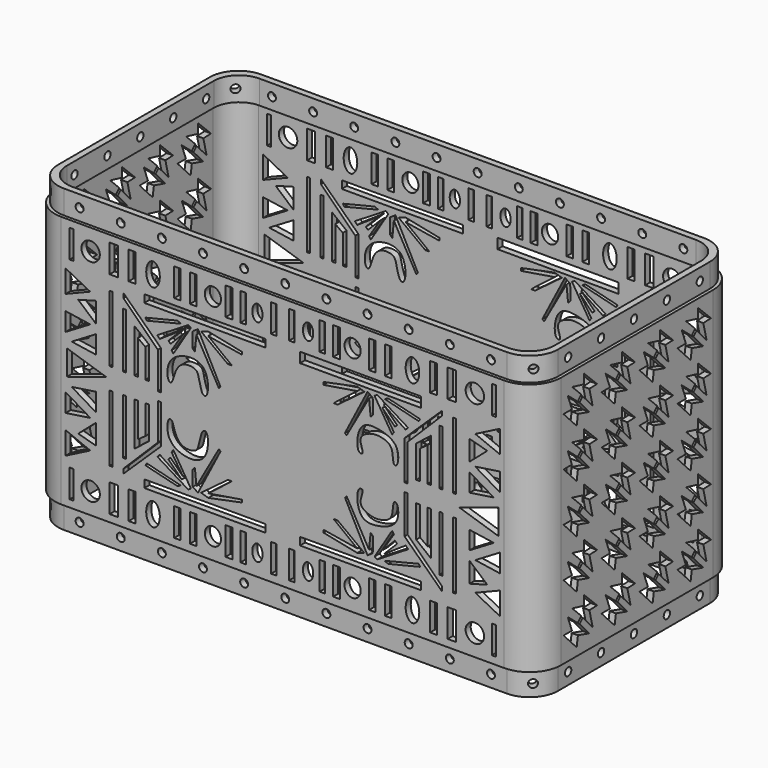
from build123d import *

# Parameters (mm, degrees)
F1_DEPTH  = 101.6
F2_T      = -2.54
F4_DEPTH  = 9.525
F6_DEPTH  = 9.525
F8_W      = 1.27
F8_H      = 26.6622491181
F8_H_2    = 22.2469121218
F8_W_2    = 48.6389496364
F8_H_3    = 3.0932202935
F8_H_4    = 4.0642395616
F8_H_5    = 0.0183284283
F8_H_6    = 3.0748918653
F8_W_3    = 1.6330480576
F8_H_7    = 11.2412478775
F8_R      = 3.7023981113
F8_W_4    = 3.2661110163
F8_W_5    = 2.7217492461
F8_W_6    = 2.6040747762
F8_W_7    = 2.5893896818
F8_W_8    = 2.1774070337
F8_W_9    = 2.7217566967
F8_W_10   = 2.1774061024
F9_DEPTH  = 127
F10_R     = 1.5875
F11_DEPTH = 127
F13_DEPTH = 228.6
F14_R     = 1.5875
F15_DEPTH = 228.6
F17_R     = 1.5875
F18_DEPTH = 50.8
F21_R     = 1.5875
F22_DEPTH = 50.8
F24_R     = 1.5875
F25_DEPTH = 76.2
F27_R     = 1.5875
F28_DEPTH = 76.2


with BuildPart() as f1:
    # F0 (on Top) → F1 (new body)
    with BuildSketch(Plane.XY):
        with BuildLine():
            Line((88.9, 50.8), (-88.9, 50.8))
            ThreePointArc((-88.9, 50.8), (-97.8802561211, 47.0802561211), (-101.6, 38.1))
            Line((-101.6, 38.1), (-101.6, -38.1))
            ThreePointArc((-101.6, -38.1), (-97.8802561211, -47.0802561211), (-88.9, -50.8))
            Line((-88.9, -50.8), (88.9, -50.8))
            ThreePointArc((88.9, -50.8), (97.8802561211, -47.0802561211), (101.6, -38.1))
            Line((101.6, -38.1), (101.6, 38.1))
            ThreePointArc((101.6, 38.1), (97.8802561211, 47.0802561211), (88.9, 50.8))
        make_face()
    extrude(amount=F1_DEPTH)

    # F2
    f2_openings = [f1.faces().sort_by_distance(p)[0] for p in [
        (0, 0, 101.6),
        (0, 0, 0),
    ]]
    offset(amount=F2_T, openings=f2_openings)

    # F3 (on face) → F4 (join)
    with BuildSketch(Plane.XY.offset(101.6)):
        with BuildLine():
            Line((-88.9, -49.53), (88.9, -49.53))
            ThreePointArc((88.9, -49.53), (96.982230509, -46.182230509), (100.33, -38.1))
            Line((100.33, -38.1), (100.33, 38.1))
            ThreePointArc((100.33, 38.1), (96.982230509, 46.182230509), (88.9, 49.53))
            Line((88.9, 49.53), (-88.9, 49.53))
            ThreePointArc((-88.9, 49.53), (-96.982230509, 46.182230509), (-100.33, 38.1))
            Line((-100.33, 38.1), (-100.33, -38.1))
            ThreePointArc((-100.33, -38.1), (-96.982230509, -46.182230509), (-88.9, -49.53))
        make_face()
        with BuildLine():
            ThreePointArc((-99.06, 38.1), (-96.0842048969, 45.2842048969), (-88.9, 48.26))
            Line((-88.9, 48.26), (88.9, 48.26))
            ThreePointArc((88.9, 48.26), (96.0842048969, 45.2842048969), (99.06, 38.1))
            Line((99.06, 38.1), (99.06, -38.1))
            ThreePointArc((99.06, -38.1), (96.0842048969, -45.2842048969), (88.9, -48.26))
            Line((88.9, -48.26), (-88.9, -48.26))
            ThreePointArc((-88.9, -48.26), (-96.0842048969, -45.2842048969), (-99.06, -38.1))
            Line((-99.06, -38.1), (-99.06, 38.1))
        make_face(mode=Mode.SUBTRACT)
        with BuildLine():
            Line((88.9, 48.26), (-88.9, 48.26))
            ThreePointArc((-88.9, 48.26), (-96.0842048969, 45.2842048969), (-99.06, 38.1))
            Line((-99.06, 38.1), (-99.06, -38.1))
            ThreePointArc((-99.06, -38.1), (-96.0842048969, -45.2842048969), (-88.9, -48.26))
            Line((-88.9, -48.26), (88.9, -48.26))
            ThreePointArc((88.9, -48.26), (96.0842048969, -45.2842048969), (99.06, -38.1))
            Line((99.06, -38.1), (99.06, 38.1))
            ThreePointArc((99.06, 38.1), (96.0842048969, 45.2842048969), (88.9, 48.26))
        make_face()
        with BuildLine():
            ThreePointArc((-97.79, 36.83), (-94.8142048969, 44.0142048969), (-87.63, 46.99))
            Line((-87.63, 46.99), (87.63, 46.99))
            ThreePointArc((87.63, 46.99), (94.8142048969, 44.0142048969), (97.79, 36.83))
            Line((97.79, 36.83), (97.79, -36.83))
            ThreePointArc((97.79, -36.83), (94.8142048969, -44.0142048969), (87.63, -46.99))
            Line((87.63, -46.99), (-87.63, -46.99))
            ThreePointArc((-87.63, -46.99), (-94.8142048969, -44.0142048969), (-97.79, -36.83))
            Line((-97.79, -36.83), (-97.79, 36.83))
        make_face(mode=Mode.SUBTRACT)
    extrude(amount=F4_DEPTH)

    # F5 (on Top) → F6 (join)
    with BuildSketch(Plane.XY):
        with BuildLine():
            Line((88.9, 49.53), (-88.9, 49.53))
            ThreePointArc((-88.9, 49.53), (-96.982230509, 46.182230509), (-100.33, 38.1))
            Line((-100.33, 38.1), (-100.33, -38.1))
            ThreePointArc((-100.33, -38.1), (-96.982230509, -46.182230509), (-88.9, -49.53))
            Line((-88.9, -49.53), (88.9, -49.53))
            ThreePointArc((88.9, -49.53), (96.982230509, -46.182230509), (100.33, -38.1))
            Line((100.33, -38.1), (100.33, 38.1))
            ThreePointArc((100.33, 38.1), (96.982230509, 46.182230509), (88.9, 49.53))
        make_face()
        with BuildLine():
            Line((87.63, -46.99), (-87.63, -46.99))
            ThreePointArc((-87.63, -46.99), (-94.8142048969, -44.0142048969), (-97.79, -36.83))
            Line((-97.79, -36.83), (-97.79, 36.83))
            ThreePointArc((-97.79, 36.83), (-94.8142048969, 44.0142048969), (-87.63, 46.99))
            Line((-87.63, 46.99), (87.63, 46.99))
            ThreePointArc((87.63, 46.99), (94.8142048969, 44.0142048969), (97.79, 36.83))
            Line((97.79, 36.83), (97.79, -36.83))
            ThreePointArc((97.79, -36.83), (94.8142048969, -44.0142048969), (87.63, -46.99))
        make_face(mode=Mode.SUBTRACT)
    extrude(amount=-F6_DEPTH)

    # F8 (on face) → F9 (cut)
    with BuildSketch(Plane.XZ.offset(50.8)):
        with Locations((-68.9020286703, 68.476928398)):
            Rectangle(F8_W, F8_H)
        with Locations((-63.4877477384, 66.1137998104)):
            Rectangle(F8_W, F8_H_2)
        Polygon((-59.5282502472, 72.5896432996), (-59.5282502472, 55.0722591579), (-58.1557303667, 55.0722591579), (-58.1557303667, 68.7985643744), (-55.1492646337, 66.6415765882), (-55.1492646337, 55.0068952143), (-53.5806752741, 55.0068952143), (-53.5806752741, 67.883476615), align=None)
        Polygon((-50.1429028809, 67.2847032547), (-50.1429028809, 52.5627210736), (-48.8572530448, 52.5627210736), (-48.8572530448, 68.2254508138), (-63.9233589172, 82.7843993902), (-63.9233589172, 80.9818580747), align=None)
        with Locations((-31.2301132362, 83.5803337395)):
            Rectangle(F8_W_2, F8_H_3)
        Polygon((-42.2406457365, 80.1282450557), (-55.1029518247, 76.9830867648), (-54.5800887048, 76.0679990053), (-40.8993884921, 79.4538781047), align=None)
        Polygon((-37.9368662834, 79.9399539828), (-50.3318198025, 72.3422840238), (-49.3153783607, 71.3319868494), (-40.5374765396, 77.2372558713), (-45.9055488806, 71.8365368266), (-45.039238331, 70.9754630211), (-40.0128401816, 76.0324299335), (-44.6069753195, 68.9266495444), (-43.8944920897, 67.867577076), (-36.8599989183, 79.27594897), align=None)
        Polygon((-36.1134645205, 78.3830672404), (-36.279860884, 72.3422840238), (-35.2634194421, 71.3319868494), (-34.6407592297, 77.6337906718), (-25.6241530731, 61.6211524411), (-24.9729361385, 62.2763298452), (-34.0206585824, 79.7909870744), align=None)
        Polygon((-32.7727422118, 79.3707743287), (-22.0318287611, 71.3319868494), (-20.3978791833, 71.3319868494), (-29.9133080989, 78.6741450429), (-16.3456853479, 76.4601826668), (-16.3456853479, 77.5059908628), (-29.8969931901, 80.269522965), align=None)
        with BuildLine():
            add(Edge.make_bspline(
                [(-45.6465967, 57.64246732), (-46.3949852869, 58.5152129663), (-46.8754204882, 65.0704943716), (-39.4761129722, 69.4554491147), (-29.7425350447, 68.3388211569), (-29.6427188035, 56.9346913808), (-32.7583018207, 56.9375001196), (-33.6608195324, 63.7843708703), (-35.1035222126, 65.6981368237), (-40.3177607972, 66.1274931074), (-43.3679070085, 62.1610139174), (-44.150056881, 57.2996314955), (-45.3474051799, 57.2935602133), (-45.6465967, 57.64246732)],
                knots=[0, 0, 0, 0, 0.1046718898, 0.2236520347, 0.3429708219, 0.4678825728, 0.5171800771, 0.6233463725, 0.6881859742, 0.7762207213, 0.869134302, 0.9581541697, 1, 1, 1, 1], degree=3))
        make_face()
        Polygon((49.3153783607, 71.3319868494), (50.3318198025, 72.3422840238), (37.9368662834, 79.9399539828), (36.8599989183, 79.27594897), (43.8944920897, 67.867577076), (44.6069753195, 68.9266495444), (40.0128401816, 76.0324299335), (45.039238331, 70.9754630211), (45.9055488806, 71.8365368266), (40.5374765396, 77.2372558713), align=None)
        Polygon((50.1429028809, 67.2847032547), (63.9233589172, 80.9818580747), (63.9233589172, 82.7843993902), (48.8572530448, 68.2254508138), (48.8572530448, 52.5627210736), (50.1429028809, 52.5627210736), align=None)
        Polygon((58.1557303667, 55.0722591579), (59.5282502472, 55.0722591579), (59.5282502472, 72.5896432996), (53.5806752741, 67.883476615), (53.5806752741, 55.0068952143), (55.1492646337, 55.0068952143), (55.1492646337, 66.6415765882), (58.1557303667, 68.7985643744), align=None)
        with Locations((31.2301132362, 83.0948241055)):
            Rectangle(F8_W_2, F8_H_4)
        Polygon((35.2634194421, 71.3319868494), (36.279860884, 72.3422840238), (36.1134645205, 78.3830672404), (34.0206585824, 79.7909870744), (24.9729361385, 62.2763298452), (25.6241530731, 61.6211524411), (34.6407592297, 77.6337906718), align=None)
        Polygon((32.7727422118, 79.3707743287), (29.8969931901, 80.269522965), (16.3456853479, 77.5059908628), (16.3456853479, 76.4601826668), (29.9133080989, 78.6741450429), (20.3978791833, 71.3319868494), (22.0318287611, 71.3319868494), align=None)
        with Locations((63.4877477384, 66.1137998104)):
            Rectangle(F8_W, F8_H_2)
        with Locations((68.9020286703, 68.476928398)):
            Rectangle(F8_W, F8_H)
        Polygon((40.8993884921, 79.4538781047), (54.5800887048, 76.0679990053), (55.1029518247, 76.9830867648), (42.2406457365, 80.1282450557), align=None)
        with BuildLine():
            add(Edge.make_bspline(
                [(45.6465967, 57.64246732), (46.4635562257, 58.5803284783), (47.0830188738, 65.3489604803), (38.5305633944, 68.4932132602), (29.9974402873, 68.4019397724), (29.3300401803, 56.8501614014), (33.1351567804, 57.0444987502), (29.5108019941, 62.8747584858), (35.5677572547, 65.8582939635), (39.6837091755, 65.677942821), (44.6266519892, 63.8299183013), (43.9427154071, 57.1850526299), (45.319991823, 57.2675282703), (45.6465967, 57.64246732)],
                knots=[0, 0, 0, 0, 0.1027137574, 0.2221431268, 0.3325537808, 0.4551287654, 0.5035040447, 0.5937830457, 0.688394598, 0.7747824494, 0.8625292723, 0.9589369938, 1, 1, 1, 1], degree=3))
        make_face()
        Polygon((-48.8572530448, 33.5269491862), (-48.8572530448, 49.1896789264), (-50.1429028809, 49.1896789264), (-50.1429028809, 34.4676967453), (-63.9233589172, 20.7705419253), (-63.9233589172, 18.9680006098), align=None)
        Polygon((-53.5806752741, 33.868923385), (-53.5806752741, 46.7455047857), (-55.1492646337, 46.7455047857), (-55.1492646337, 35.1108234118), (-58.1557303667, 32.9538356256), (-58.1557303667, 46.6801408421), (-59.5282502472, 46.6801408421), (-59.5282502472, 29.1627567004), align=None)
        with Locations((-63.4877477384, 35.6386001896)):
            Rectangle(F8_W, F8_H_2)
        with Locations((-68.9020286703, 33.275471602)):
            Rectangle(F8_W, F8_H)
        Polygon((-36.1134645205, 23.3693327596), (-34.0206585824, 21.9614129256), (-24.9729361385, 39.4760701548), (-25.6241530731, 40.1312475589), (-34.6407592297, 24.1186093282), (-35.2634194421, 30.4204131506), (-36.279860884, 29.4101159762), align=None)
        Polygon((-32.7727422118, 22.3816256713), (-29.8969931901, 21.482877035), (-16.3456853479, 24.2464091372), (-16.3456853479, 25.2922173332), (-29.9133080989, 23.0782549571), (-20.3978791833, 30.4204131506), (-22.0318287611, 30.4204131506), align=None)
        Polygon((-49.3153783607, 30.4204131506), (-50.3318198025, 29.4101159762), (-37.9368662834, 21.8124460172), (-36.8599989183, 22.47645103), (-43.8944920897, 33.884822924), (-44.6069753195, 32.8257504556), (-40.0128401816, 25.7199700665), (-45.039238331, 30.7769369789), (-45.9055488806, 29.9158631734), (-40.5374765396, 24.5151441287), align=None)
        with Locations((-31.2301132362, 19.7095121931)):
            Rectangle(F8_W_2, F8_H_5)
        with Locations((-31.2301132362, 18.1629020463)):
            Rectangle(F8_W_2, F8_H_6)
        Polygon((-55.1029518247, 24.7693132352), (-42.2406457365, 21.6241549443), (-40.8993884921, 22.2985218953), (-54.5800887048, 25.6844009947), align=None)
        with BuildLine():
            add(Edge.make_bspline(
                [(-45.6465967, 44.10993268), (-46.3949852869, 43.2371870337), (-46.8754204882, 36.6819056284), (-39.4761129722, 32.2969508853), (-29.7425350447, 33.4135788431), (-29.6427188035, 44.8177086192), (-32.7583018207, 44.8148998804), (-33.6608195324, 37.9680291297), (-35.1035222126, 36.0542631763), (-40.3177607972, 35.6249068926), (-43.3679070085, 39.5913860826), (-44.150056881, 44.4527685045), (-45.3474051799, 44.4588397867), (-45.6465967, 44.10993268)],
                knots=[0, 0, 0, 0, 0.1046718898, 0.2236520347, 0.3429708219, 0.4678825728, 0.5171800771, 0.6233463725, 0.6881859742, 0.7762207213, 0.869134302, 0.9581541697, 1, 1, 1, 1], degree=3))
        make_face()
        with Locations((63.4877477384, 35.6386001896)):
            Rectangle(F8_W, F8_H_2)
        Polygon((24.9729361385, 39.4760701548), (34.0206585824, 21.9614129256), (36.1134645205, 23.3693327596), (36.279860884, 29.4101159762), (35.2634194421, 30.4204131506), (34.6407592297, 24.1186093282), (25.6241530731, 40.1312475589), align=None)
        Polygon((40.8993884921, 22.2985218953), (42.2406457365, 21.6241549443), (55.1029518247, 24.7693132352), (54.5800887048, 25.6844009947), align=None)
        Polygon((37.9368662834, 21.8124460172), (50.3318198025, 29.4101159762), (49.3153783607, 30.4204131506), (40.5374765396, 24.5151441287), (45.9055488806, 29.9158631734), (45.039238331, 30.7769369789), (40.0128401816, 25.7199700665), (44.6069753195, 32.8257504556), (43.8944920897, 33.884822924), (36.8599989183, 22.47645103), align=None)
        with Locations((68.9020286703, 33.275471602)):
            Rectangle(F8_W, F8_H)
        Polygon((29.9133080989, 23.0782549571), (16.3456853479, 25.2922173332), (16.3456853479, 24.2464091372), (29.8969931901, 21.482877035), (32.7727422118, 22.3816256713), (22.0318287611, 30.4204131506), (20.3978791833, 30.4204131506), align=None)
        Polygon((58.1557303667, 32.9538356256), (55.1492646337, 35.1108234118), (55.1492646337, 46.7455047857), (53.5806752741, 46.7455047857), (53.5806752741, 33.868923385), (59.5282502472, 29.1627567004), (59.5282502472, 46.6801408421), (58.1557303667, 46.6801408421), align=None)
        Polygon((63.9233589172, 18.9680006098), (63.9233589172, 20.7705419253), (50.1429028809, 34.4676967453), (50.1429028809, 49.1896789264), (48.8572530448, 49.1896789264), (48.8572530448, 33.5269491862), align=None)
        with Locations((31.2301132362, 18.1629020463)):
            Rectangle(F8_W_2, F8_H_6)
        with Locations((31.2301132362, 19.7095121931)):
            Rectangle(F8_W_2, F8_H_5)
        with BuildLine():
            add(Edge.make_bspline(
                [(45.6465967, 44.10993268), (46.4635562257, 43.1720715217), (47.0830188738, 36.4034395197), (38.5305633944, 33.2591867398), (29.9974402873, 33.3504602276), (29.3300401803, 44.9022385986), (33.1351567804, 44.7079012498), (29.5108019941, 38.8776415142), (35.5677572547, 35.8941060365), (39.6837091755, 36.074457179), (44.6266519892, 37.9224816987), (43.9427154071, 44.5673473701), (45.319991823, 44.4848717297), (45.6465967, 44.10993268)],
                knots=[0, 0, 0, 0, 0.1027137574, 0.2221431268, 0.3325537808, 0.4551287654, 0.5035040447, 0.5937830457, 0.688394598, 0.7747824494, 0.8625292723, 0.9589369938, 1, 1, 1, 1], degree=3))
        make_face()
        with Locations((-84.7257450223, 8.5211573169)):
            Rectangle(F8_W_3, F8_H_7)
        with Locations((-77.1048292518, 8.5211573169)):
            Circle(F8_R)
        with Locations((-67.8508579731, 8.5211573169)):
            Rectangle(F8_W_4, F8_H_7)
        with Locations((-60.5021193624, 8.5211573169)):
            Rectangle(F8_W_5, F8_H_7)
        with BuildLine():
            add(Edge.make_bspline(
                [(-52.0646758378, 13.1481420249), (-56.7870740248, 13.1481420249), (-54.4258749313, 6.2076649629), (-52.0646758378, -0.7328120992), (-49.7034767442, 6.2076649629), (-47.3422776507, 13.1481420249), (-52.0646758378, 13.1481420249)],
                knots=[0, 0, 0, 2.0943951024, 2.0943951024, 4.1887902048, 4.1887902048, 6.2831853072, 6.2831853072, 6.2831853072], degree=2, weights=[1, 0.5, 1, 0.5, 1, 0.5, 1]))
        make_face()
        with Locations((-42.2663539648, 8.5211573169)):
            Rectangle(F8_W_6, F8_H_7)
        with Locations((-35.9620712698, 8.5211573169)):
            Rectangle(F8_W_7, F8_H_7)
        with BuildLine():
            add(Edge.make_bspline(
                [(-28.0320812017, 12.0741277933), (-33.6435658598, 12.0741277933), (-30.8378235307, 6.7446720786), (-28.0320812017, 1.415216364), (-25.2263388726, 6.7446720786), (-22.4205965436, 12.0741277933), (-28.0320812017, 12.0741277933)],
                knots=[0, 0, 0, 2.0943951024, 2.0943951024, 4.1887902048, 4.1887902048, 6.2831853072, 6.2831853072, 6.2831853072], degree=2, weights=[1, 0.5, 1, 0.5, 1, 0.5, 1]))
        make_face()
        with Locations((-3.6404510029, 8.5211573169)):
            Rectangle(F8_W_8, F8_H_7)
        with BuildLine():
            add(Edge.make_bspline(
                [(-10.1726669818, 11.7913372815), (-13.7381730329, 11.7913372815), (-11.9554200073, 6.8860673346), (-10.1726669818, 1.9807973877), (-8.3899139563, 6.8860673346), (-6.6071609308, 11.7913372815), (-10.1726669818, 11.7913372815)],
                knots=[0, 0, 0, 2.0943951024, 2.0943951024, 4.1887902048, 4.1887902048, 6.2831853072, 6.2831853072, 6.2831853072], degree=2, weights=[1, 0.5, 1, 0.5, 1, 0.5, 1]))
        make_face()
        with Locations((-21.604038775, 8.5211573169)):
            Rectangle(F8_W_9, F8_H_7)
        with Locations((-15.8883500844, 8.5211573169)):
            Rectangle(F8_W_10, F8_H_7)
        with Locations((84.7257450223, 8.5211573169)):
            Rectangle(F8_W_3, F8_H_7)
        with Locations((15.8883500844, 8.5211573169)):
            Rectangle(F8_W_10, F8_H_7)
        with Locations((35.9620712698, 8.5211573169)):
            Rectangle(F8_W_7, F8_H_7)
        with Locations((42.2663539648, 8.5211573169)):
            Rectangle(F8_W_6, F8_H_7)
        with Locations((21.604038775, 8.5211573169)):
            Rectangle(F8_W_9, F8_H_7)
        with Locations((67.8508579731, 8.5211573169)):
            Rectangle(F8_W_4, F8_H_7)
        with Locations((3.6404510029, 8.5211573169)):
            Rectangle(F8_W_8, F8_H_7)
        with Locations((60.5021193624, 8.5211573169)):
            Rectangle(F8_W_5, F8_H_7)
        with BuildLine():
            add(Edge.make_bspline(
                [(52.0646758378, 13.1481420249), (47.3422776507, 13.1481420249), (49.7034767442, 6.2076649629), (52.0646758378, -0.7328120992), (54.4258749313, 6.2076649629), (56.7870740248, 13.1481420249), (52.0646758378, 13.1481420249)],
                knots=[0, 0, 0, 2.0943951024, 2.0943951024, 4.1887902048, 4.1887902048, 6.2831853072, 6.2831853072, 6.2831853072], degree=2, weights=[1, 0.5, 1, 0.5, 1, 0.5, 1]))
        make_face()
        with BuildLine():
            add(Edge.make_bspline(
                [(10.1726669818, 11.7913372815), (6.6071609308, 11.7913372815), (8.3899139563, 6.8860673346), (10.1726669818, 1.9807973877), (11.9554200073, 6.8860673346), (13.7381730329, 11.7913372815), (10.1726669818, 11.7913372815)],
                knots=[0, 0, 0, 2.0943951024, 2.0943951024, 4.1887902048, 4.1887902048, 6.2831853072, 6.2831853072, 6.2831853072], degree=2, weights=[1, 0.5, 1, 0.5, 1, 0.5, 1]))
        make_face()
        with Locations((77.1048292518, 8.5211573169)):
            Circle(F8_R)
        with BuildLine():
            add(Edge.make_bspline(
                [(28.0320812017, 12.0741277933), (22.4205965436, 12.0741277933), (25.2263388726, 6.7446720786), (28.0320812017, 1.415216364), (30.8378235307, 6.7446720786), (33.6435658598, 12.0741277933), (28.0320812017, 12.0741277933)],
                knots=[0, 0, 0, 2.0943951024, 2.0943951024, 4.1887902048, 4.1887902048, 6.2831853072, 6.2831853072, 6.2831853072], degree=2, weights=[1, 0.5, 1, 0.5, 1, 0.5, 1]))
        make_face()
        with Locations((84.7257450223, 93.2312426831)):
            Rectangle(F8_W_3, F8_H_7)
        with Locations((3.6404510029, 93.2312426831)):
            Rectangle(F8_W_8, F8_H_7)
        with Locations((-42.2663539648, 93.2312426831)):
            Rectangle(F8_W_6, F8_H_7)
        with Locations((15.8883500844, 93.2312426831)):
            Rectangle(F8_W_10, F8_H_7)
        with Locations((42.2663539648, 93.2312426831)):
            Rectangle(F8_W_6, F8_H_7)
        with Locations((21.604038775, 93.2312426831)):
            Rectangle(F8_W_9, F8_H_7)
        with Locations((-15.8883500844, 93.2312426831)):
            Rectangle(F8_W_10, F8_H_7)
        with Locations((-60.5021193624, 93.2312426831)):
            Rectangle(F8_W_5, F8_H_7)
        with Locations((-67.8508579731, 93.2312426831)):
            Rectangle(F8_W_4, F8_H_7)
        with Locations((60.5021193624, 93.2312426831)):
            Rectangle(F8_W_5, F8_H_7)
        with Locations((67.8508579731, 93.2312426831)):
            Rectangle(F8_W_4, F8_H_7)
        with Locations((35.9620712698, 93.2312426831)):
            Rectangle(F8_W_7, F8_H_7)
        with Locations((-3.6404510029, 93.2312426831)):
            Rectangle(F8_W_8, F8_H_7)
        with Locations((-35.9620712698, 93.2312426831)):
            Rectangle(F8_W_7, F8_H_7)
        with Locations((-21.604038775, 93.2312426831)):
            Rectangle(F8_W_9, F8_H_7)
        with Locations((-84.7257450223, 93.2312426831)):
            Rectangle(F8_W_3, F8_H_7)
        with BuildLine():
            add(Edge.make_bspline(
                [(10.1726669818, 89.9610627185), (13.7381730329, 89.9610627185), (11.9554200073, 94.8663326654), (10.1726669818, 99.7716026123), (8.3899139563, 94.8663326654), (6.6071609308, 89.9610627185), (10.1726669818, 89.9610627185)],
                knots=[0, 0, 0, 2.0943951024, 2.0943951024, 4.1887902048, 4.1887902048, 6.2831853072, 6.2831853072, 6.2831853072], degree=2, weights=[1, 0.5, 1, 0.5, 1, 0.5, 1]))
        make_face()
        with BuildLine():
            add(Edge.make_bspline(
                [(-28.0320812017, 89.6782722067), (-22.4205965436, 89.6782722067), (-25.2263388726, 95.0077279214), (-28.0320812017, 100.337183636), (-30.8378235307, 95.0077279214), (-33.6435658598, 89.6782722067), (-28.0320812017, 89.6782722067)],
                knots=[0, 0, 0, 2.0943951024, 2.0943951024, 4.1887902048, 4.1887902048, 6.2831853072, 6.2831853072, 6.2831853072], degree=2, weights=[1, 0.5, 1, 0.5, 1, 0.5, 1]))
        make_face()
        with BuildLine():
            add(Edge.make_bspline(
                [(52.0646758378, 88.6042579751), (56.7870740248, 88.6042579751), (54.4258749313, 95.5447350371), (52.0646758378, 102.4852120992), (49.7034767442, 95.5447350371), (47.3422776507, 88.6042579751), (52.0646758378, 88.6042579751)],
                knots=[0, 0, 0, 2.0943951024, 2.0943951024, 4.1887902048, 4.1887902048, 6.2831853072, 6.2831853072, 6.2831853072], degree=2, weights=[1, 0.5, 1, 0.5, 1, 0.5, 1]))
        make_face()
        with Locations((77.1048292518, 93.2312426831)):
            Circle(F8_R)
        with BuildLine():
            add(Edge.make_bspline(
                [(28.0320812017, 89.6782722067), (33.6435658598, 89.6782722067), (30.8378235307, 95.0077279214), (28.0320812017, 100.337183636), (25.2263388726, 95.0077279214), (22.4205965436, 89.6782722067), (28.0320812017, 89.6782722067)],
                knots=[0, 0, 0, 2.0943951024, 2.0943951024, 4.1887902048, 4.1887902048, 6.2831853072, 6.2831853072, 6.2831853072], degree=2, weights=[1, 0.5, 1, 0.5, 1, 0.5, 1]))
        make_face()
        with BuildLine():
            add(Edge.make_bspline(
                [(-52.0646758378, 88.6042579751), (-47.3422776507, 88.6042579751), (-49.7034767442, 95.5447350371), (-52.0646758378, 102.4852120992), (-54.4258749313, 95.5447350371), (-56.7870740248, 88.6042579751), (-52.0646758378, 88.6042579751)],
                knots=[0, 0, 0, 2.0943951024, 2.0943951024, 4.1887902048, 4.1887902048, 6.2831853072, 6.2831853072, 6.2831853072], degree=2, weights=[1, 0.5, 1, 0.5, 1, 0.5, 1]))
        make_face()
        with BuildLine():
            add(Edge.make_bspline(
                [(-10.1726669818, 89.9610627185), (-6.6071609308, 89.9610627185), (-8.3899139563, 94.8663326654), (-10.1726669818, 99.7716026123), (-11.9554200073, 94.8663326654), (-13.7381730329, 89.9610627185), (-10.1726669818, 89.9610627185)],
                knots=[0, 0, 0, 2.0943951024, 2.0943951024, 4.1887902048, 4.1887902048, 6.2831853072, 6.2831853072, 6.2831853072], degree=2, weights=[1, 0.5, 1, 0.5, 1, 0.5, 1]))
        make_face()
        with Locations((-77.1048292518, 93.2312426831)):
            Circle(F8_R)
        Polygon((-77.2655457258, 78.9374113083), (-87.1297195554, 83.9744359255), (-87.1297195554, 74.9497637153), align=None)
        Polygon((-75.0258415937, 68.4268182709), (-75.0258415937, 76.4573417283), (-82.0926949382, 74.5300129056), align=None)
        Polygon((-77.2655457258, 67.3942267895), (-87.1297195554, 68.8633620739), (-87.1297195554, 61.5176968277), align=None)
        Polygon((-75.0258415937, 57.4427627866), (-75.0258415937, 64.6428851634), (-84.6945722448, 58.8827894529), align=None)
        Polygon((-86.6621136665, 55.9206530452), (-86.6621136665, 50.8762), (-86.6621136665, 45.8317469548), (-70.8759278059, 50.8762), align=None)
        Polygon((-75.0258415937, 37.1095148366), (-75.0258415937, 44.3096372134), (-84.6945722448, 42.8696105471), align=None)
        Polygon((-87.1297195554, 32.8890379261), (-77.2655457258, 34.3581732105), (-87.1297195554, 40.2347031723), align=None)
        Polygon((-87.1297195554, 17.7779640745), (-77.2655457258, 22.8149886917), (-87.1297195554, 26.8026362847), align=None)
        Polygon((-82.0926949382, 27.2223870944), (-75.0258415937, 25.2950582717), (-75.0258415937, 33.3255817291), align=None)
        Polygon((70.8759278059, 50.8762), (86.6621136665, 45.8317469548), (86.6621136665, 50.8762), (86.6621136665, 55.9206530452), align=None)
        Polygon((75.0258415937, 44.3096372134), (75.0258415937, 37.1095148366), (84.6945722448, 42.8696105471), align=None)
        Polygon((75.0258415937, 33.3255817291), (75.0258415937, 25.2950582717), (82.0926949382, 27.2223870944), align=None)
        Polygon((77.2655457258, 67.3942267895), (87.1297195554, 61.5176968277), (87.1297195554, 68.8633620739), align=None)
        Polygon((75.0258415937, 68.4268182709), (82.0926949382, 74.5300129056), (75.0258415937, 76.4573417283), align=None)
        Polygon((87.1297195554, 17.7779640745), (87.1297195554, 26.8026362847), (77.2655457258, 22.8149886917), align=None)
        Polygon((75.0258415937, 64.6428851634), (75.0258415937, 57.4427627866), (84.6945722448, 58.8827894529), align=None)
        Polygon((77.2655457258, 34.3581732105), (87.1297195554, 32.8890379261), (87.1297195554, 40.2347031723), align=None)
        Polygon((87.1297195554, 83.9744359255), (77.2655457258, 78.9374113083), (87.1297195554, 74.9497637153), align=None)
    extrude(amount=-F9_DEPTH, mode=Mode.SUBTRACT)

    # F10 (on face) → F11 (cut)
    with BuildSketch(Plane.XZ.offset(49.53)):
        with Locations((0, 106.3625)):
            Circle(F10_R)
        with Locations((-16.51, 106.3625)):
            Circle(F10_R)
        with Locations((-33.02, 106.3625)):
            Circle(F10_R)
        with Locations((-49.53, 106.3625)):
            Circle(F10_R)
        with Locations((-66.04, 106.3625)):
            Circle(F10_R)
        with Locations((-82.55, 106.3625)):
            Circle(F10_R)
        with Locations((16.51, 106.3625)):
            Circle(F10_R)
        with Locations((33.02, 106.3625)):
            Circle(F10_R)
        with Locations((49.53, 106.3625)):
            Circle(F10_R)
        with Locations((66.04, 106.3625)):
            Circle(F10_R)
        with Locations((82.55, 106.3625)):
            Circle(F10_R)
        with Locations((82.55, -4.7625)):
            Circle(F10_R)
        with Locations((66.04, -4.7625)):
            Circle(F10_R)
        with Locations((49.53, -4.7625)):
            Circle(F10_R)
        with Locations((33.02, -4.7625)):
            Circle(F10_R)
        with Locations((16.51, -4.7625)):
            Circle(F10_R)
        with Locations((0, -4.7625)):
            Circle(F10_R)
        with Locations((-16.51, -4.7625)):
            Circle(F10_R)
        with Locations((-33.02, -4.7625)):
            Circle(F10_R)
        with Locations((-49.53, -4.7625)):
            Circle(F10_R)
        with Locations((-66.04, -4.7625)):
            Circle(F10_R)
        with Locations((-82.55, -4.7625)):
            Circle(F10_R)
    extrude(amount=-F11_DEPTH, mode=Mode.SUBTRACT)

    # F12 (on face) → F13 (cut)
    with BuildSketch(Plane(origin=(-101.6, 0, 0), x_dir=(0, -1, 0), z_dir=(-1, 0, 0))):
        Polygon((-30.5271521211, 98.34882617), (-37.0560400188, 92.0305550098), (-33.1948697567, 91.8901413679), (-34.82172117, 85.1895782738), (-29.8476629601, 90.5899843302), (-28.2104499638, 89.0820249915), (-33.124666661, 83.7465897202), (-27.4382159114, 85.3612571955), (-26.8063880503, 81.3596844673), (-20.2345553491, 88.2172510028), (-24.4455895363, 88.2172510028), (-22.3133917898, 93.9260348678), (-27.3455451271, 89.7338111294), (-29.1230902076, 91.5391296148), (-24.5598908514, 96.032127738), (-30.5271521211, 94.5578664541), align=None)
        Polygon((-28.2104499638, 69.5240249915), (-33.124666661, 64.1885897202), (-27.4382159114, 65.8032571955), (-26.8063880503, 61.8016844673), (-20.2345553491, 68.6592510028), (-24.4455895363, 68.6592510028), (-22.3133917898, 74.3680348678), (-27.3455451271, 70.1758111294), (-29.1230902076, 71.9811296148), (-24.5598908514, 76.474127738), (-30.5271521211, 74.9998664541), (-30.5271521211, 78.79082617), (-37.0560400188, 72.4725550098), (-33.1948697567, 72.3321413679), (-34.82172117, 65.6315782738), (-29.8476629601, 71.0319843302), align=None)
        Polygon((-28.2104499638, 49.9660249915), (-33.124666661, 44.6305897202), (-27.4382159114, 46.2452571955), (-26.8063880503, 42.2436844673), (-20.2345553491, 49.1012510028), (-24.4455895363, 49.1012510028), (-22.3133917898, 54.8100348678), (-27.3455451271, 50.6178111294), (-29.1230902076, 52.4231296148), (-24.5598908514, 56.916127738), (-30.5271521211, 55.4418664541), (-30.5271521211, 59.23282617), (-37.0560400188, 52.9145550098), (-33.1948697567, 52.7741413679), (-34.82172117, 46.0735782738), (-29.8476629601, 51.4739843302), align=None)
        Polygon((-28.2104499638, 30.4080249915), (-33.124666661, 25.0725897202), (-27.4382159114, 26.6872571955), (-26.8063880503, 22.6856844673), (-20.2345553491, 29.5432510028), (-24.4455895363, 29.5432510028), (-22.3133917898, 35.2520348678), (-27.3455451271, 31.0598111294), (-29.1230902076, 32.8651296148), (-24.5598908514, 37.358127738), (-30.5271521211, 35.8838664541), (-30.5271521211, 39.67482617), (-37.0560400188, 33.3565550098), (-33.1948697567, 33.2161413679), (-34.82172117, 26.5155782738), (-29.8476629601, 31.9159843302), align=None)
        Polygon((-9.1604499638, 89.0820249915), (-14.074666661, 83.7465897202), (-8.3882159114, 85.3612571955), (-7.7563880503, 81.3596844673), (-1.1845553491, 88.2172510028), (-5.3955895363, 88.2172510028), (-3.2633917898, 93.9260348678), (-8.2955451271, 89.7338111294), (-10.0730902076, 91.5391296148), (-5.5098908514, 96.032127738), (-11.4771521211, 94.5578664541), (-11.4771521211, 98.34882617), (-18.0060400188, 92.0305550098), (-14.1448697567, 91.8901413679), (-15.77172117, 85.1895782738), (-10.7976629601, 90.5899843302), align=None)
        Polygon((-9.1604499638, 69.5240249915), (-14.074666661, 64.1885897202), (-8.3882159114, 65.8032571955), (-7.7563880503, 61.8016844673), (-1.1845553491, 68.6592510028), (-5.3955895363, 68.6592510028), (-3.2633917898, 74.3680348678), (-8.2955451271, 70.1758111294), (-10.0730902076, 71.9811296148), (-5.5098908514, 76.474127738), (-11.4771521211, 74.9998664541), (-11.4771521211, 78.79082617), (-18.0060400188, 72.4725550098), (-14.1448697567, 72.3321413679), (-15.77172117, 65.6315782738), (-10.7976629601, 71.0319843302), align=None)
        Polygon((-9.1604499638, 49.9660249915), (-14.074666661, 44.6305897202), (-8.3882159114, 46.2452571955), (-7.7563880503, 42.2436844673), (-1.1845553491, 49.1012510028), (-5.3955895363, 49.1012510028), (-3.2633917898, 54.8100348678), (-8.2955451271, 50.6178111294), (-10.0730902076, 52.4231296148), (-5.5098908514, 56.916127738), (-11.4771521211, 55.4418664541), (-11.4771521211, 59.23282617), (-18.0060400188, 52.9145550098), (-14.1448697567, 52.7741413679), (-15.77172117, 46.0735782738), (-10.7976629601, 51.4739843302), align=None)
        Polygon((-9.1604499638, 30.4080249915), (-14.074666661, 25.0725897202), (-8.3882159114, 26.6872571955), (-7.7563880503, 22.6856844673), (-1.1845553491, 29.5432510028), (-5.3955895363, 29.5432510028), (-3.2633917898, 35.2520348678), (-8.2955451271, 31.0598111294), (-10.0730902076, 32.8651296148), (-5.5098908514, 37.358127738), (-11.4771521211, 35.8838664541), (-11.4771521211, 39.67482617), (-18.0060400188, 33.3565550098), (-14.1448697567, 33.2161413679), (-15.77172117, 26.5155782738), (-10.7976629601, 31.9159843302), align=None)
        Polygon((9.8895500362, 89.0820249915), (4.975333339, 83.7465897202), (10.6617840886, 85.3612571955), (11.2936119497, 81.3596844673), (17.8654446509, 88.2172510028), (13.6544104637, 88.2172510028), (15.7866082102, 93.9260348678), (10.7544548729, 89.7338111294), (8.9769097924, 91.5391296148), (13.5401091486, 96.032127738), (7.5728478789, 94.5578664541), (7.5728478789, 98.34882617), (1.0439599812, 92.0305550098), (4.9051302433, 91.8901413679), (3.27827883, 85.1895782738), (8.2523370399, 90.5899843302), align=None)
        Polygon((9.8895500362, 69.5240249915), (4.975333339, 64.1885897202), (10.6617840886, 65.8032571955), (11.2936119497, 61.8016844673), (17.8654446509, 68.6592510028), (13.6544104637, 68.6592510028), (15.7866082102, 74.3680348678), (10.7544548729, 70.1758111294), (8.9769097924, 71.9811296148), (13.5401091486, 76.474127738), (7.5728478789, 74.9998664541), (7.5728478789, 78.79082617), (1.0439599812, 72.4725550098), (4.9051302433, 72.3321413679), (3.27827883, 65.6315782738), (8.2523370399, 71.0319843302), align=None)
        Polygon((9.8895500362, 49.9660249915), (4.975333339, 44.6305897202), (10.6617840886, 46.2452571955), (11.2936119497, 42.2436844673), (17.8654446509, 49.1012510028), (13.6544104637, 49.1012510028), (15.7866082102, 54.8100348678), (10.7544548729, 50.6178111294), (8.9769097924, 52.4231296148), (13.5401091486, 56.916127738), (7.5728478789, 55.4418664541), (7.5728478789, 59.23282617), (1.0439599812, 52.9145550098), (4.9051302433, 52.7741413679), (3.27827883, 46.0735782738), (8.2523370399, 51.4739843302), align=None)
        Polygon((9.8895500362, 30.4080249915), (4.975333339, 25.0725897202), (10.6617840886, 26.6872571955), (11.2936119497, 22.6856844673), (17.8654446509, 29.5432510028), (13.6544104637, 29.5432510028), (15.7866082102, 35.2520348678), (10.7544548729, 31.0598111294), (8.9769097924, 32.8651296148), (13.5401091486, 37.358127738), (7.5728478789, 35.8838664541), (7.5728478789, 39.67482617), (1.0439599812, 33.3565550098), (4.9051302433, 33.2161413679), (3.27827883, 26.5155782738), (8.2523370399, 31.9159843302), align=None)
        Polygon((28.9395500362, 89.0820249915), (24.025333339, 83.7465897202), (29.7117840886, 85.3612571955), (30.3436119497, 81.3596844673), (36.9154446509, 88.2172510028), (32.7044104637, 88.2172510028), (34.8366082102, 93.9260348678), (29.8044548729, 89.7338111294), (28.0269097924, 91.5391296148), (32.5901091486, 96.032127738), (26.6228478789, 94.5578664541), (26.6228478789, 98.34882617), (20.0939599812, 92.0305550098), (23.9551302433, 91.8901413679), (22.32827883, 85.1895782738), (27.3023370399, 90.5899843302), align=None)
        Polygon((28.9395500362, 69.5240249915), (24.025333339, 64.1885897202), (29.7117840886, 65.8032571955), (30.3436119497, 61.8016844673), (36.9154446509, 68.6592510028), (32.7044104637, 68.6592510028), (34.8366082102, 74.3680348678), (29.8044548729, 70.1758111294), (28.0269097924, 71.9811296148), (32.5901091486, 76.474127738), (26.6228478789, 74.9998664541), (26.6228478789, 78.79082617), (20.0939599812, 72.4725550098), (23.9551302433, 72.3321413679), (22.32827883, 65.6315782738), (27.3023370399, 71.0319843302), align=None)
        Polygon((28.9395500362, 49.9660249915), (24.025333339, 44.6305897202), (29.7117840886, 46.2452571955), (30.3436119497, 42.2436844673), (36.9154446509, 49.1012510028), (32.7044104637, 49.1012510028), (34.8366082102, 54.8100348678), (29.8044548729, 50.6178111294), (28.0269097924, 52.4231296148), (32.5901091486, 56.916127738), (26.6228478789, 55.4418664541), (26.6228478789, 59.23282617), (20.0939599812, 52.9145550098), (23.9551302433, 52.7741413679), (22.32827883, 46.0735782738), (27.3023370399, 51.4739843302), align=None)
        Polygon((28.9395500362, 30.4080249915), (24.025333339, 25.0725897202), (29.7117840886, 26.6872571955), (30.3436119497, 22.6856844673), (36.9154446509, 29.5432510028), (32.7044104637, 29.5432510028), (34.8366082102, 35.2520348678), (29.8044548729, 31.0598111294), (28.0269097924, 32.8651296148), (32.5901091486, 37.358127738), (26.6228478789, 35.8838664541), (26.6228478789, 39.67482617), (20.0939599812, 33.3565550098), (23.9551302433, 33.2161413679), (22.32827883, 26.5155782738), (27.3023370399, 31.9159843302), align=None)
        Polygon((-28.2104499638, 10.8500249915), (-33.124666661, 5.5145897202), (-27.4382159114, 7.1292571955), (-26.8063880503, 3.1276844673), (-20.2345553491, 9.9852510028), (-24.4455895363, 9.9852510028), (-22.3133917898, 15.6940348678), (-27.3455451271, 11.5018111294), (-29.1230902076, 13.3071296148), (-24.5598908514, 17.800127738), (-30.5271521211, 16.3258664541), (-30.5271521211, 20.11682617), (-37.0560400188, 13.7985550098), (-33.1948697567, 13.6581413679), (-34.82172117, 6.9575782738), (-29.8476629601, 12.3579843302), align=None)
        Polygon((-9.1604499638, 10.8500249915), (-14.074666661, 5.5145897202), (-8.3882159114, 7.1292571955), (-7.7563880503, 3.1276844673), (-1.1845553491, 9.9852510028), (-5.3955895363, 9.9852510028), (-3.2633917898, 15.6940348678), (-8.2955451271, 11.5018111294), (-10.0730902076, 13.3071296148), (-5.5098908514, 17.800127738), (-11.4771521211, 16.3258664541), (-11.4771521211, 20.11682617), (-18.0060400188, 13.7985550098), (-14.1448697567, 13.6581413679), (-15.77172117, 6.9575782738), (-10.7976629601, 12.3579843302), align=None)
        Polygon((9.8895500362, 10.8500249915), (4.975333339, 5.5145897202), (10.6617840886, 7.1292571955), (11.2936119497, 3.1276844673), (17.8654446509, 9.9852510028), (13.6544104637, 9.9852510028), (15.7866082102, 15.6940348678), (10.7544548729, 11.5018111294), (8.9769097924, 13.3071296148), (13.5401091486, 17.800127738), (7.5728478789, 16.3258664541), (7.5728478789, 20.11682617), (1.0439599812, 13.7985550098), (4.9051302433, 13.6581413679), (3.27827883, 6.9575782738), (8.2523370399, 12.3579843302), align=None)
        Polygon((28.9395500362, 10.8500249915), (24.025333339, 5.5145897202), (29.7117840886, 7.1292571955), (30.3436119497, 3.1276844673), (36.9154446509, 9.9852510028), (32.7044104637, 9.9852510028), (34.8366082102, 15.6940348678), (29.8044548729, 11.5018111294), (28.0269097924, 13.3071296148), (32.5901091486, 17.800127738), (26.6228478789, 16.3258664541), (26.6228478789, 20.11682617), (20.0939599812, 13.7985550098), (23.9551302433, 13.6581413679), (22.32827883, 6.9575782738), (27.3023370399, 12.3579843302), align=None)
    extrude(amount=-F13_DEPTH, mode=Mode.SUBTRACT)

    # F14 (on face) → F15 (cut)
    with BuildSketch(Plane.YZ.offset(100.33)):
        with Locations((0, 106.3625)):
            Circle(F14_R)
        with Locations((-16.51, 106.3625)):
            Circle(F14_R)
        with Locations((16.51, 106.3625)):
            Circle(F14_R)
        with Locations((-33.02, 106.3625)):
            Circle(F14_R)
        with Locations((33.02, 106.3625)):
            Circle(F14_R)
        with Locations((33.02, -4.7625)):
            Circle(F14_R)
        with Locations((16.51, -4.7625)):
            Circle(F14_R)
        with Locations((0, -4.7625)):
            Circle(F14_R)
        with Locations((-16.51, -4.7625)):
            Circle(F14_R)
        with Locations((-33.02, -4.7625)):
            Circle(F14_R)
    extrude(amount=-F15_DEPTH, mode=Mode.SUBTRACT)

    # F17 (on face) → F18 (cut)
    with BuildSketch(Plane(origin=(63.5, -63.5, 0), x_dir=(-0.7071067812, -0.7071067812, 0), z_dir=(-0.7071067812, 0.7071067812, 0))):
        with Locations((-35.7487341389, -4.7304881737)):
            Circle(F17_R)
        with Locations((-35.9213575721, 106.4095161855)):
            Circle(F17_R)
    extrude(amount=-F18_DEPTH, mode=Mode.SUBTRACT)

    # F21 (on face) → F22 (cut)
    with BuildSketch(Plane(origin=(-63.5, -63.5, 0), x_dir=(0.7071067812, -0.7071067812, 0), z_dir=(-0.7071067812, -0.7071067812, 0))):
        with Locations((-35.9600037336, -4.758330062)):
            Circle(F21_R)
        with Locations((-35.9600037336, 106.4215265214)):
            Circle(F21_R)
    extrude(amount=F22_DEPTH, mode=Mode.SUBTRACT)

    # F24 (on face) → F25 (cut)
    with BuildSketch(Plane(origin=(-62.223585695, 62.223585695, 0), x_dir=(-0.7071067812, -0.7071067812, 0), z_dir=(-0.7071067812, 0.7071067812, 0))):
        with Locations((35.9291117638, -4.7214720398)):
            Circle(F24_R)
        with Locations((35.9291117638, 106.4158603549)):
            Circle(F24_R)
    extrude(amount=F25_DEPTH, mode=Mode.SUBTRACT)

    # F27 (on face) → F28 (cut)
    with BuildSketch(Plane(origin=(62.223585695, 62.223585695, 0), x_dir=(0.7071067812, -0.7071067812, 0), z_dir=(-0.7071067812, -0.7071067812, 0))):
        with Locations((35.9206516296, 106.4431853592)):
            Circle(F27_R)
        with Locations((35.9206516296, -4.7728870995)):
            Circle(F27_R)
    extrude(amount=-F28_DEPTH, mode=Mode.SUBTRACT)


solid = f1.part
